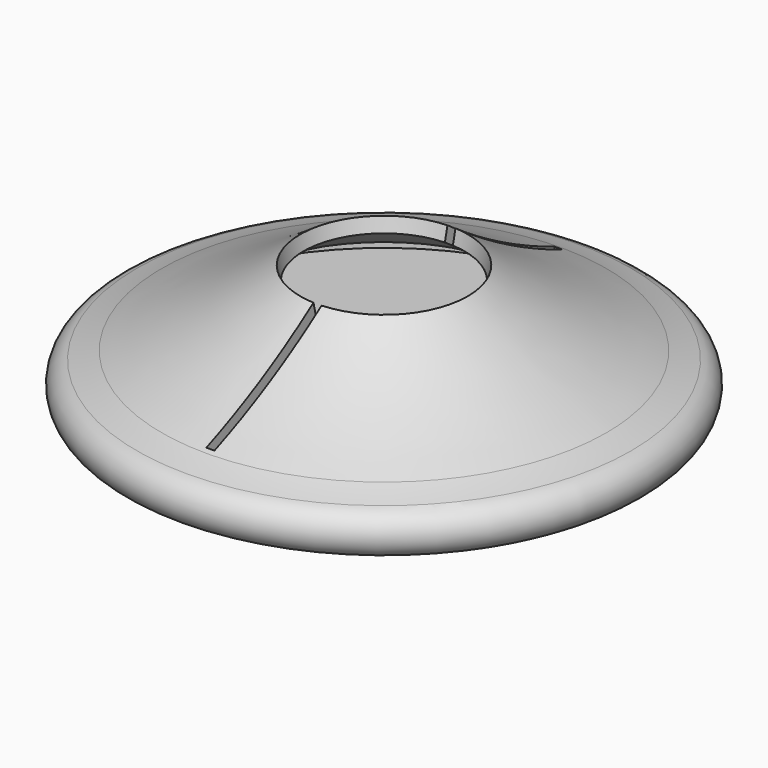
from build123d import *

# Parameters (mm, degrees)
F3_R     = 25
F5_START = -2.7
F4_W     = 1
F4_H     = 53.9998769996
F5_DEPTH = 22.3


# Not quite as in the source:
# - a fillet or chamfer that OpenCascade refuses, or shapes differently, is made with other operations: its cross-section is extruded or revolved along the edge and cut away or added


with BuildPart() as f1:
    # F0 (on Front) → F1 (revolve)
    with BuildSketch(Plane.XZ):
        with BuildLine():
            ThreePointArc((3, 1), (12.6231681205, -4.9677750086), (23, -9.5))
            Line((23, -9.5), (23, -11))
            Line((23, -11), (-7, -11))
            Line((-7, -11), (-7, -13))
            Line((-7, -13), (23, -13))
            ThreePointArc((23, -13), (25.75, -10.25), (23, -7.5))
            ThreePointArc((23, -7.5), (12.6231681205, -2.9677750086), (3, 3))
            Line((3, 3), (3, 1))
        make_face()
    revolve(axis=Axis((-7, 0, -1.698827371), (0, 0, -1)))

    # F2: chamfer of 0.5 x 2 on 1 edges, made by hand

    # F2_s1 → F2_t2 (revolve, cut)
    with BuildSketch(Plane.XZ):
        with BuildLine():
            Line((3.4123952329, 2.7941574241), (2.9820609835, 0.9239297508))
            Line((2.9820609835, 0.9239297508), (2.9420609835, 0.9239297508))
            ThreePointArc((2.9420609835, 0.9239297508), (2.96, 1.9619648754), (2.96, 3))
            Line((2.96, 3), (3.0234608243, 3.0323973722))
            ThreePointArc((3.0234608243, 3.0323973722), (3.2078025867, 2.8993085114), (3.4356565384, 2.8266983471))
            Line((3.4356565384, 2.8266983471), (3.4123952329, 2.7941574241))
        make_face()
    revolve(axis=Axis((-7, 0, 3), (0, 0, -1)), mode=Mode.SUBTRACT)

    # F3
    f3_edges = [f1.edges().sort_by_distance(p)[0] for p in [
        (-37, 0, -7.5),
    ]]
    fillet(f3_edges, radius=F3_R)

    # F4 (on face) → F5 (cut)
    with BuildSketch(Plane(origin=(0, 0, -13), x_dir=(1, 0, 0), z_dir=(0, 0, -1)).offset(F5_START)):
        with Locations((-6.9392545743, 0)):
            Rectangle(F4_W, F4_H)
    extrude(amount=-F5_DEPTH, mode=Mode.SUBTRACT)


solid = f1.part
